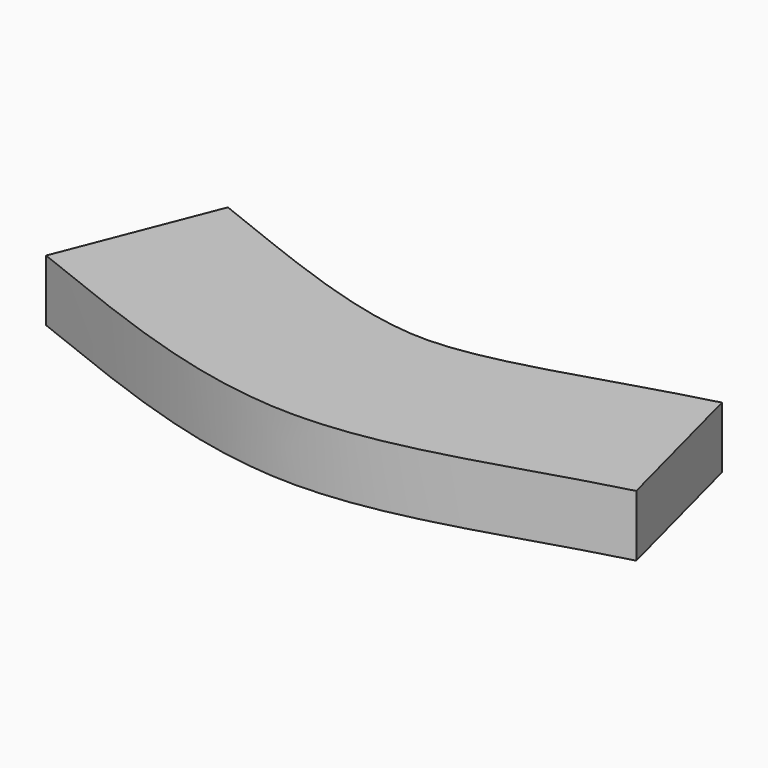
from build123d import *

# Parameters (mm, degrees)
F1_DEPTH = 19.05


# Not quite as in the source:
# - the dataset's text gives a spline's control points without its knots; the knots are read off the source's solid


with BuildPart() as f1:
    # F0 (on Top) → F1 (new body)
    with BuildSketch(Plane.XY):
        with BuildLine():
            Line((-78.7400000139, 74.9710454241), (-97.3307817617, 27.6950173125))
            add(Edge.make_bspline(
                [(-97.3307817617, 27.6950173125), (-66.2225142701, 15.4620308585), (0.5303698628, -13.9302166383), (60.3542314066, 12.4911491454), (91.5026097765, 20.5759386309)],
                knots=[0, 0, 0, 0, 0.5095002534, 1, 1, 1, 1], degree=3))
            Line((91.5026097765, 20.5759386309), (78.74, 69.7466188346))
            add(Edge.make_bspline(
                [(-78.7400000139, 74.9710454241), (-74.751639175, 73.4026660815), (-66.8993742503, 70.2653188702), (-55.4971155584, 65.7379336533), (-44.5182059311, 61.5615862051), (-34.0480869505, 57.8985675644), (-25.8469948752, 55.3948961673), (-19.6753333366, 53.7774059809), (-15.2618679349, 52.7661333276), (-11.084222746, 51.9627067048), (-7.1622127924, 51.3683727178), (-4.121108692, 51.0441951948), (-1.8312034682, 50.8828940784), (-0.4592915947, 50.8215137555), (0.6000811821, 50.7951820381), (1.6422815166, 50.7835190193), (2.9793902335, 50.7954852513), (4.6264900218, 50.8533409822), (6.3249262074, 50.9554896058), (8.076907396, 51.1028768126), (10.4883899189, 51.3608560651), (13.6498371919, 51.8005785667), (17.6904338769, 52.5196453595), (21.9827064774, 53.4296073156), (26.5274721813, 54.5252716267), (32.9220353822, 56.2200505467), (41.5374163561, 58.7426199425), (52.8616329275, 62.2529894112), (65.1868389817, 66.0273969194), (74.0997387513, 68.5422050796), (78.74, 69.7466188346)],
                knots=[0, 0, 0, 0, 0.0625, 0.125, 0.1875, 0.25, 0.3125, 0.34375, 0.375, 0.40625, 0.4375, 0.46875, 0.484375, 0.5, 0.5078125, 0.515625, 0.53125, 0.546875, 0.5625, 0.578125, 0.59375, 0.625, 0.65625, 0.6875, 0.71875, 0.75, 0.8125, 0.875, 0.9375, 1, 1, 1, 1], degree=3))
        make_face()
    extrude(amount=F1_DEPTH)


solid = f1.part
